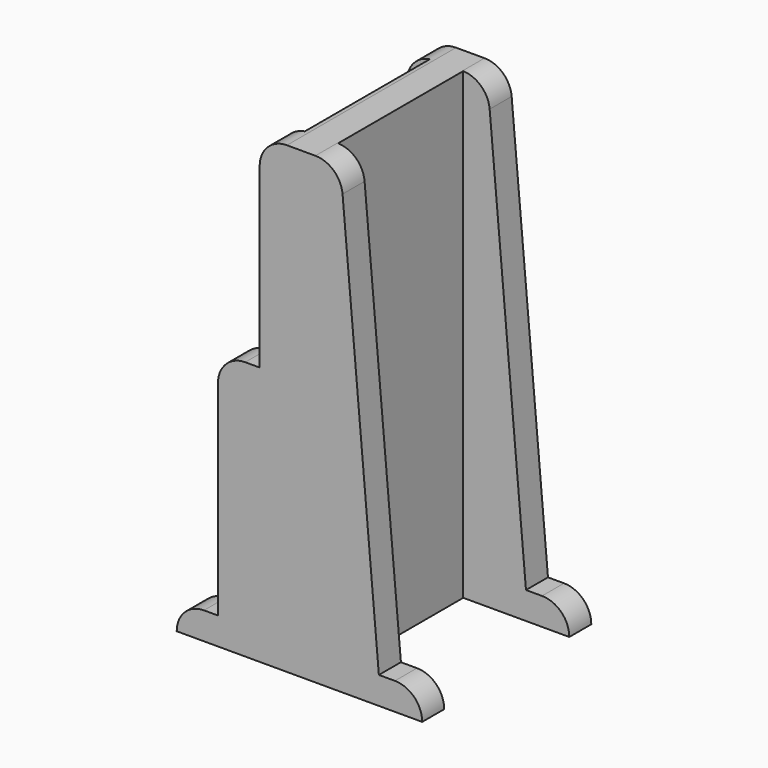
from build123d import *

# Parameters (mm, degrees)
F0_W        = 3.0256015398
F0_H        = 2.0134245381
F1_DEPTH    = 2
F0_W_2      = 3.0003240481
F0_H_2      = 2.0157374777
F0_H_3      = 2.019865565
F0_W_3      = 3.0242641605
F2_DEPTH    = 34
F3_DEPTH    = 34
F0_W_4      = 3.0575518031
F0_W_5      = 3.0562144239
F4_DEPTH    = 19
F5_T4_DEPTH = 178.7945589271
F5_T9_DEPTH = 178.7904308398
F7_F1_R     = 1.9999
F7_F2_R     = 1.9999
F7_F3_R     = 1.9999
F7_F4_R     = 1.9999
F7_F5_R     = 2
F7_F6_R     = 2
F7_F7_R     = 2
F8_F1_R     = 2


# Not quite as in the source:
# - a fillet or chamfer that OpenCascade refuses, or shapes differently, is made with other operations: its cross-section is extruded or revolved along the edge and cut away or added
# - two fillets or chamfers of one size are made in one step
# - a fillet or chamfer is up to 0.001 mm smaller than in the source, because OpenCascade refuses the exact size


with BuildPart() as f1:
    # F0 (on Top) → F1 (new body)
    with BuildSketch(Plane.XY):
        with Locations((-7.4871992301, 6.743287731)):
            Rectangle(F0_W, F0_H)
    extrude(amount=F1_DEPTH)



with BuildPart() as f1b:
    # F0 (on Top) → F1, piece 2 (new body)
    with BuildSketch(Plane.XY):
        with Locations((7.4998379759, 6.7421312612)):
            Rectangle(F0_W_2, F0_H_2)
    extrude(amount=F1_DEPTH)



with BuildPart() as f1c:
    # F0 (on Top) → F1, piece 3 (new body)
    with BuildSketch(Plane.XY):
        with Locations((7.4998379759, -6.7400672175)):
            Rectangle(F0_W_2, F0_H_3)
    extrude(amount=F1_DEPTH)


with BuildPart() as f1d:
    # F0 (on Top) → F1, piece 4 (new body)
    with BuildSketch(Plane.XY):
        with Locations((-7.4878679197, -6.7400672175)):
            Rectangle(F0_W_3, F0_H_3)
    extrude(amount=F1_DEPTH)


with BuildPart() as f2:
    # F0 (on Top) → F2 (new body)
    with BuildSketch(Plane.XY):
        Polygon((1.2222049991, -5.730134435), (1.2222049991, 5.7342625223), (1.2222049991, 7.5), (-1.2222049991, 7.5), (-1.2222049991, 5.7365754619), (-1.2222049991, -5.730134435), (-1.2222049991, -7.5), (1.2222049991, -7.5), align=None)
    extrude(amount=F2_DEPTH)


with BuildPart() as f1b_1:
    add(f1b.part)

    add(f1c.part)  # F3 merges F1c

    add(f2.part)  # F3 merges F2
    # F0 (on Top) → F3 (join)
    with BuildSketch(Plane.XY):
        Polygon((5.9996759519, 5.7342625223), (5.9996759519, 7.75), (-2.9181840364, 7.75), (-2.9181840364, 5.7365754619), (-1.2222049991, 5.7365754619), (-1.2222049991, 7.5), (1.2222049991, 7.5), (1.2222049991, 5.7342625223), align=None)
        Polygon((5.9996759519, -7.75), (5.9996759519, -5.730134435), (1.2222049991, -5.730134435), (1.2222049991, -7.5), (-1.2222049991, -7.5), (-1.2222049991, -5.730134435), (-2.9181840364, -5.730134435), (-2.9181840364, -7.75), align=None)
    extrude(amount=F3_DEPTH)


with BuildPart() as f1_1:
    add(f1.part)

    add(f1b_1.part)  # F4 merges F1b

    add(f1d.part)  # F4 merges F1d
    # F0 (on Top) → F4 (join)
    with BuildSketch(Plane.XY):
        with Locations((-4.4469599379, -6.7400672175)):
            Rectangle(F0_W_4, F0_H_3)
        with Locations((-4.4462912483, 6.743287731)):
            Rectangle(F0_W_5, F0_H)
    extrude(amount=F4_DEPTH)

    # F5: chamfer of 3 x 34 on 2 edges, made by hand


with BuildPart() as f5_tool2:
    # F5_s3 → F5_t4 (new body)
    with BuildSketch(Plane.XZ.offset(96.137346681)):
        Polygon((5.9996759519, 0), (2.9996759519, 34), (5.9996759519, 34), align=None)
    extrude(amount=-F5_T4_DEPTH)

    split(bisect_by=Plane.XY.offset(2), keep=Keep.TOP)


with BuildPart() as f1_2:
    add(f1_1.part)

    # F5_t1: cut F5_tool2
    add(f5_tool2.part, mode=Mode.SUBTRACT)


with BuildPart() as f5_tool7:
    # F5_s8 → F5_t9 (new body)
    with BuildSketch(Plane.XZ.offset(82.6530841587)):
        Polygon((5.9996759519, 0), (2.9996759519, 34), (5.9996759519, 34), align=None)
    extrude(amount=-F5_T9_DEPTH)

    split(bisect_by=Plane.XY.offset(2), keep=Keep.TOP)


with BuildPart() as f1_3:
    add(f1_2.part)

    # F5_t6: cut F5_tool7
    add(f5_tool7.part, mode=Mode.SUBTRACT)

    # F7: fillet of radius 2 on 8 edges, made by hand

    # F7_f1 (radius 2 in the source; OpenCascade refuses exactly that, so slightly less here)
    f7_f1_edges = [f1_3.edges().sort_by_distance(p)[0] for p in [
        (-9, -6.7400672175, 2),
    ]]
    fillet(f7_f1_edges, radius=F7_F1_R)

    # F7_f2 (radius 2 in the source; OpenCascade refuses exactly that, so slightly less here)
    f7_f2_edges = [f1_3.edges().sort_by_distance(p)[0] for p in [
        (9, -6.7400672175, 2),
    ]]
    fillet(f7_f2_edges, radius=F7_F2_R)

    # F7_f3 (radius 2 in the source; OpenCascade refuses exactly that, so slightly less here)
    f7_f3_edges = [f1_3.edges().sort_by_distance(p)[0] for p in [
        (9, 6.7421312612, 2),
    ]]
    fillet(f7_f3_edges, radius=F7_F3_R)

    # F7_f4 (radius 2 in the source; OpenCascade refuses exactly that, so slightly less here)
    f7_f4_edges = [f1_3.edges().sort_by_distance(p)[0] for p in [
        (-9, 6.743287731, 2),
    ]]
    fillet(f7_f4_edges, radius=F7_F4_R)

    # F7_f5
    f7_f5_edges = [f1_3.edges().sort_by_distance(p)[0] for p in [
        (-5.9743984602, 6.743287731, 19),
    ]]
    fillet(f7_f5_edges, radius=F7_F5_R)

    # F7_f6
    f7_f6_edges = [f1_3.edges().sort_by_distance(p)[0] for p in [
        (-2.9181840364, 6.743287731, 34),
    ]]
    fillet(f7_f6_edges, radius=F7_F6_R)

    # F7_f7
    f7_f7_edges = [f1_3.edges().sort_by_distance(p)[0] for p in [
        (-5.9757358395, -6.7400672175, 19),
    ]]
    fillet(f7_f7_edges, radius=F7_F7_R)

    # F8: fillet of radius 2 on 2 edges, made by hand

    # F8_f1
    f8_f1_edges = [f1_3.edges().sort_by_distance(p)[0] for p in [
        (2.9996759519, -6.7400672175, 34),
    ]]
    fillet(f8_f1_edges, radius=F8_F1_R)


solid = f1_3.part
